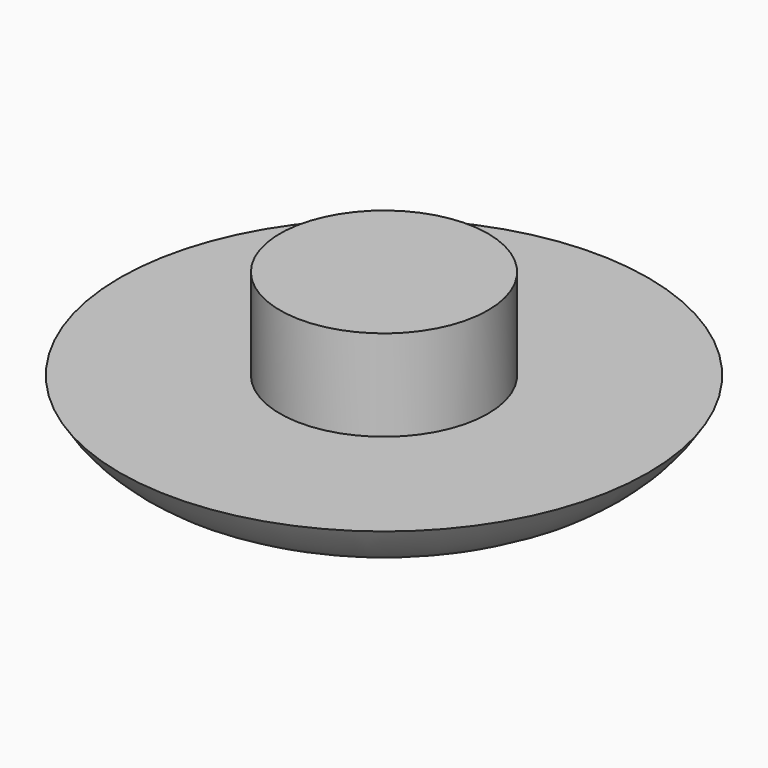
from build123d import *

# Parameters (mm, degrees)
F0_R     = 10.16
F1_DEPTH = 2.5
F2_R     = 4
F3_DEPTH = 3.5


# Not quite as in the source:
# - a fillet or chamfer that OpenCascade refuses, or shapes differently, is made with other operations: its cross-section is extruded or revolved along the edge and cut away or added


with BuildPart() as f1:
    # F0 (on Top) → F1 (new body)
    with BuildSketch(Plane.XY):
        Circle(F0_R)
    extrude(amount=F1_DEPTH)

    # F2 (on face) → F3 (join)
    with BuildSketch(Plane.XY.offset(2.5)):
        Circle(F2_R)
    extrude(amount=F3_DEPTH)

    # F4: fillet of radius 5 on 1 edges, made by hand

    # F4_s1 → F4_t2 (revolve, cut)
    with BuildSketch(Plane.XZ):
        with BuildLine():
            ThreePointArc((10.16, 2.5), (8.3298729811, 0.6698729811), (5.8298729811, 0))
            Line((5.8298729811, 0), (10.16, 0))
            Line((10.16, 0), (10.16, 2.5))
        make_face()
    revolve(axis=Axis((0, 0, 0), (0, 0, 1)), mode=Mode.SUBTRACT)


solid = f1.part
